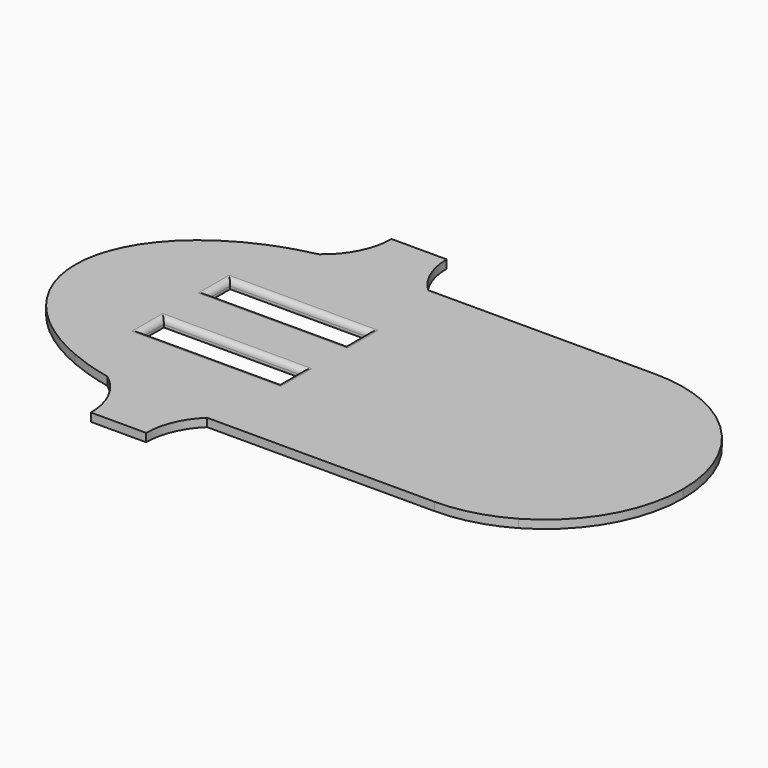
from build123d import *

# Parameters (mm, degrees)
F1_DEPTH = 3
F2_R     = 2
F3_DEPTH = 2


with BuildPart() as f1:
    # F0 (on Top) → F1 (new body)
    with BuildSketch(Plane.XY):
        with BuildLine():
            add(Edge.make_bspline(
                [(0, 0), (10.2976274735, 0), (20.158993222, 2.1182632902)],
                knots=[1.5707963268, 1.5707963268, 1.5707963268, 1.8629189995, 1.8629189995, 1.8629189995], degree=2, weights=[1, 0.9893519935, 1]))
            Line((0, 0), (17.6506484271, 0))
            ThreePointArc((17.6506484271, 0), (18.8700107709, 1.1003520247), (20.158993222, 2.1182632902))
        make_face()
        with BuildLine():
            add(Edge.make_bspline(
                [(-20.158993222, 2.1182632902), (-10.2976274735, 0), (0, 0)],
                knots=[1.2786736541, 1.2786736541, 1.2786736541, 1.5707963268, 1.5707963268, 1.5707963268], degree=2, weights=[1, 0.9893519935, 1]))
            Line((0, 0), (0, 30))
            Line((0, 30), (-10, 30))
            Line((-10, 30), (-30, 30))
            Line((-30, 30), (-30, 40))
            Line((-30, 40), (-10, 40))
            Line((-10, 40), (0, 40))
            Line((0, 40), (0, 50))
            Line((0, 50), (-70, 50))
            add(Edge.make_bspline(
                [(-70, 50), (-70, 21.516086051), (-35.6976035326, 6.9902650909)],
                knots=[0, 0, 0, 1.0356513364, 1.0356513364, 1.0356513364], degree=2, weights=[1, 0.8688975097, 1]))
            ThreePointArc((-35.6976035326, 6.9902650909), (-27.5204903752, 5.8549142898), (-20.158993222, 2.1182632902))
        make_face()
        with BuildLine():
            Line((0, -18), (0, 0))
            add(Edge.make_bspline(
                [(-20.158993222, 2.1182632902), (-10.2976274735, 0), (0, 0)],
                knots=[1.2786736541, 1.2786736541, 1.2786736541, 1.5707963268, 1.5707963268, 1.5707963268], degree=2, weights=[1, 0.9893519935, 1]))
            ThreePointArc((-20.158993222, 2.1182632902), (-12.6838044298, -6.7311307011), (-10, -18))
            Line((-10, -18), (0, -18))
        make_face()
        with BuildLine():
            Line((0, 30), (0, 0))
            add(Edge.make_bspline(
                [(0, 0), (10.2976274735, 0), (20.158993222, 2.1182632902)],
                knots=[1.5707963268, 1.5707963268, 1.5707963268, 1.8629189995, 1.8629189995, 1.8629189995], degree=2, weights=[1, 0.9893519935, 1]))
            ThreePointArc((20.158993222, 2.1182632902), (27.5204903752, 5.8549142898), (35.6976035326, 6.9902650909))
            add(Edge.make_bspline(
                [(35.6976035326, 6.9902650909), (49.4779363229, 12.8257362969), (58.3333333333, 22.3614600804)],
                knots=[2.1059413172, 2.1059413172, 2.1059413172, 2.5559071101, 2.5559071101, 2.5559071101], degree=2, weights=[1, 0.9747979228, 1]))
            ThreePointArc((58.3333333333, 22.3614600804), (52.1286446122, 35.5662432703), (50, 50))
            Line((50, 50), (0, 50))
            Line((0, 50), (0, 40))
            Line((0, 40), (20, 40))
            Line((20, 40), (20, 30))
            Line((20, 30), (0, 30))
        make_face()
        with BuildLine():
            Line((17.6506484271, 0), (0, 0))
            Line((0, 0), (0, -18))
            Line((0, -18), (10, -18))
            ThreePointArc((10, -18), (11.9920254116, -8.2207819669), (17.6506484271, 0))
        make_face()
        with BuildLine():
            ThreePointArc((20.158993222, 2.1182632902), (18.8700107709, 1.1003520247), (17.6506484271, 0))
            Line((17.6506484271, 0), (52.3493515729, 0))
            ThreePointArc((52.3493515729, 0), (44.67672975, 5.0512668056), (35.6976035326, 6.9902650909))
            add(Edge.make_bspline(
                [(20.158993222, 2.1182632902), (28.3447518468, 3.8765990461), (35.6976035326, 6.9902650909)],
                knots=[1.8629189995, 1.8629189995, 1.8629189995, 2.1059413172, 2.1059413172, 2.1059413172], degree=2, weights=[1, 0.9926265982, 1]))
        make_face()
        with BuildLine():
            add(Edge.make_bspline(
                [(-35.6976035326, 6.9902650909), (-28.3447518468, 3.8765990461), (-20.158993222, 2.1182632902)],
                knots=[1.0356513364, 1.0356513364, 1.0356513364, 1.2786736541, 1.2786736541, 1.2786736541], degree=2, weights=[1, 0.9926265982, 1]))
            ThreePointArc((-20.158993222, 2.1182632902), (-27.5204903752, 5.8549142898), (-35.6976035326, 6.9902650909))
        make_face()
        with BuildLine():
            ThreePointArc((35.6976035326, 6.9902650909), (27.5204903752, 5.8549142898), (20.158993222, 2.1182632902))
            add(Edge.make_bspline(
                [(20.158993222, 2.1182632902), (28.3447518468, 3.8765990461), (35.6976035326, 6.9902650909)],
                knots=[1.8629189995, 1.8629189995, 1.8629189995, 2.1059413172, 2.1059413172, 2.1059413172], degree=2, weights=[1, 0.9926265982, 1]))
        make_face()
        with BuildLine():
            ThreePointArc((35.6976035326, 6.9902650909), (44.67672975, 5.0512668056), (52.3493515729, 0))
            Line((52.3493515729, 0), (100, 0))
            ThreePointArc((100, 0), (76.3560472423, 5.9436327191), (58.3333333333, 22.3614600804))
            add(Edge.make_bspline(
                [(35.6976035326, 6.9902650909), (49.4779363229, 12.8257362969), (58.3333333333, 22.3614600804)],
                knots=[2.1059413172, 2.1059413172, 2.1059413172, 2.5559071101, 2.5559071101, 2.5559071101], degree=2, weights=[1, 0.9747979228, 1]))
        make_face()
        with BuildLine():
            ThreePointArc((58.3333333333, 22.3614600804), (76.3560472423, 5.9436327191), (100, 0))
            ThreePointArc((100, 0), (112.9409522551, 1.7037086855), (125, 6.6987298108))
            ThreePointArc((125, 6.6987298108), (110.8310397827, 18.9227968521), (102.1486677301, 35.5))
            Line((102.1486677301, 35.5), (85.5, 35.5))
            Line((85.5, 35.5), (85.5, 50))
            Line((85.5, 50), (70, 50))
            add(Edge.make_bspline(
                [(58.3333333333, 22.3614600804), (70, 34.9244327711), (70, 50)],
                knots=[2.5559071101, 2.5559071101, 2.5559071101, 3.1415926536, 3.1415926536, 3.1415926536], degree=2, weights=[1, 0.9574271078, 1]))
        make_face()
        with BuildLine():
            add(Edge.make_bspline(
                [(-35.6976035326, 93.0097349091), (-70, 78.483913949), (-70, 50)],
                knots=[5.2475339708, 5.2475339708, 5.2475339708, 6.2831853072, 6.2831853072, 6.2831853072], degree=2, weights=[1, 0.8688975097, 1]))
            Line((-70, 50), (0, 50))
            Line((0, 50), (0, 60))
            Line((0, 60), (-10, 60))
            Line((-10, 60), (-30, 60))
            Line((-30, 60), (-30, 70))
            Line((-30, 70), (-10, 70))
            Line((-10, 70), (0, 70))
            Line((0, 70), (0, 100))
            add(Edge.make_bspline(
                [(0, 100), (-10.2976274735, 100), (-20.158993222, 97.8817367098)],
                knots=[4.7123889804, 4.7123889804, 4.7123889804, 5.0045116531, 5.0045116531, 5.0045116531], degree=2, weights=[1, 0.9893519935, 1]))
            add(Edge.make_bspline(
                [(-20.158993222, 97.8817367098), (-28.3447518468, 96.1234009539), (-35.6976035326, 93.0097349091)],
                knots=[5.0045116531, 5.0045116531, 5.0045116531, 5.2475339708, 5.2475339708, 5.2475339708], degree=2, weights=[1, 0.9926265982, 1]))
        make_face()
        with BuildLine():
            ThreePointArc((50, 50), (52.1286446122, 35.5662432703), (58.3333333333, 22.3614600804))
            add(Edge.make_bspline(
                [(58.3333333333, 22.3614600804), (70, 34.9244327711), (70, 50)],
                knots=[2.5559071101, 2.5559071101, 2.5559071101, 3.1415926536, 3.1415926536, 3.1415926536], degree=2, weights=[1, 0.9574271078, 1]))
            Line((70, 50), (50, 50))
        make_face()
        with BuildLine():
            ThreePointArc((102.1486677301, 35.5), (110.8310397827, 18.9227968521), (125, 6.6987298108))
            ThreePointArc((125, 6.6987298108), (143.3012701892, 25), (150, 50))
            Line((150, 50), (114.5, 50))
            Line((114.5, 50), (114.5, 35.5))
            Line((114.5, 35.5), (102.1486677301, 35.5))
        make_face()
        with BuildLine():
            Line((0, 60), (0, 50))
            Line((0, 50), (50, 50))
            ThreePointArc((50, 50), (52.1286446122, 64.4337567297), (58.3333333333, 77.6385399196))
            add(Edge.make_bspline(
                [(58.3333333333, 77.6385399196), (49.4779363229, 87.1742637031), (35.6976035326, 93.0097349091)],
                knots=[3.727278197, 3.727278197, 3.727278197, 4.17724399, 4.17724399, 4.17724399], degree=2, weights=[1, 0.9747979228, 1]))
            ThreePointArc((35.6976035326, 93.0097349091), (27.5204903752, 94.1450857102), (20.158993222, 97.8817367098))
            add(Edge.make_bspline(
                [(20.158993222, 97.8817367098), (10.2976274735, 100), (0, 100)],
                knots=[4.4202663077, 4.4202663077, 4.4202663077, 4.7123889804, 4.7123889804, 4.7123889804], degree=2, weights=[1, 0.9893519935, 1]))
            Line((0, 100), (0, 70))
            Line((0, 70), (20, 70))
            Line((20, 70), (20, 60))
            Line((20, 60), (0, 60))
        make_face()
        with BuildLine():
            Line((50, 50), (70, 50))
            add(Edge.make_bspline(
                [(70, 50), (70, 65.0755672289), (58.3333333333, 77.6385399196)],
                knots=[3.1415926536, 3.1415926536, 3.1415926536, 3.727278197, 3.727278197, 3.727278197], degree=2, weights=[1, 0.9574271078, 1]))
            ThreePointArc((58.3333333333, 77.6385399196), (52.1286446122, 64.4337567297), (50, 50))
        make_face()
        with BuildLine():
            add(Edge.make_bspline(
                [(70, 50), (70, 65.0755672289), (58.3333333333, 77.6385399196)],
                knots=[3.1415926536, 3.1415926536, 3.1415926536, 3.727278197, 3.727278197, 3.727278197], degree=2, weights=[1, 0.9574271078, 1]))
            Line((70, 50), (85.5, 50))
            Line((85.5, 50), (85.5, 64.5))
            Line((85.5, 64.5), (102.1486677301, 64.5))
            ThreePointArc((102.1486677301, 64.5), (110.8310397827, 81.0772031479), (125, 93.3012701892))
            ThreePointArc((125, 93.3012701892), (112.9409522551, 98.2962913145), (100, 100))
            ThreePointArc((100, 100), (76.3560472423, 94.0563672809), (58.3333333333, 77.6385399196))
        make_face()
        with BuildLine():
            Line((85.5, 35.5), (102.1486677301, 35.5))
            ThreePointArc((102.1486677301, 35.5), (101.8578009321, 36.4970866512), (101.5877081724, 37.5))
            Line((101.5877081724, 37.5), (87.5, 37.5))
            Line((87.5, 37.5), (87.5, 50))
            Line((87.5, 50), (85.5, 50))
            Line((85.5, 50), (85.5, 35.5))
        make_face()
        with BuildLine():
            ThreePointArc((101.5877081724, 37.5), (101.8578009321, 36.4970866512), (102.1486677301, 35.5))
            Line((102.1486677301, 35.5), (114.5, 35.5))
            Line((114.5, 35.5), (114.5, 50))
            Line((114.5, 50), (112.5, 50))
            Line((112.5, 50), (112.5, 37.5))
            Line((112.5, 37.5), (101.5877081724, 37.5))
        make_face()
        with BuildLine():
            Line((114.5, 50), (150, 50))
            ThreePointArc((150, 50), (143.3012701892, 75), (125, 93.3012701892))
            ThreePointArc((125, 93.3012701892), (110.8310397827, 81.0772031479), (102.1486677301, 64.5))
            Line((102.1486677301, 64.5), (114.5, 64.5))
            Line((114.5, 64.5), (114.5, 50))
        make_face()
        with BuildLine():
            ThreePointArc((-10, 118), (-12.6838044298, 106.7311307011), (-20.158993222, 97.8817367098))
            add(Edge.make_bspline(
                [(0, 100), (-10.2976274735, 100), (-20.158993222, 97.8817367098)],
                knots=[4.7123889804, 4.7123889804, 4.7123889804, 5.0045116531, 5.0045116531, 5.0045116531], degree=2, weights=[1, 0.9893519935, 1]))
            Line((0, 100), (0, 118))
            Line((0, 118), (-10, 118))
        make_face()
        with BuildLine():
            add(Edge.make_bspline(
                [(58.3333333333, 77.6385399196), (49.4779363229, 87.1742637031), (35.6976035326, 93.0097349091)],
                knots=[3.727278197, 3.727278197, 3.727278197, 4.17724399, 4.17724399, 4.17724399], degree=2, weights=[1, 0.9747979228, 1]))
            ThreePointArc((58.3333333333, 77.6385399196), (76.3560472423, 94.0563672809), (100, 100))
            Line((100, 100), (52.3493515729, 100))
            ThreePointArc((52.3493515729, 100), (44.67672975, 94.9487331944), (35.6976035326, 93.0097349091))
        make_face()
        with BuildLine():
            Line((85.5, 64.5), (85.5, 50))
            Line((85.5, 50), (87.5, 50))
            Line((87.5, 50), (87.5, 62.5))
            Line((87.5, 62.5), (101.5877081724, 62.5))
            ThreePointArc((101.5877081724, 62.5), (101.8578009321, 63.5029133488), (102.1486677301, 64.5))
            Line((102.1486677301, 64.5), (85.5, 64.5))
        make_face()
        with BuildLine():
            Line((87.5, 37.5), (101.5877081724, 37.5))
            ThreePointArc((101.5877081724, 37.5), (100.3985151866, 43.6997853759), (100, 50))
            Line((100, 50), (87.5, 50))
            Line((87.5, 50), (87.5, 37.5))
        make_face()
        with BuildLine():
            ThreePointArc((100, 50), (100.3985151866, 43.6997853759), (101.5877081724, 37.5))
            Line((101.5877081724, 37.5), (112.5, 37.5))
            Line((112.5, 37.5), (112.5, 50))
            Line((112.5, 50), (100, 50))
        make_face()
        with BuildLine():
            Line((112.5, 50), (114.5, 50))
            Line((114.5, 50), (114.5, 64.5))
            Line((114.5, 64.5), (102.1486677301, 64.5))
            ThreePointArc((102.1486677301, 64.5), (101.8578009321, 63.5029133488), (101.5877081724, 62.5))
            Line((101.5877081724, 62.5), (112.5, 62.5))
            Line((112.5, 62.5), (112.5, 50))
        make_face()
        with BuildLine():
            Line((0, 118), (0, 100))
            Line((0, 100), (17.6506484271, 100))
            ThreePointArc((17.6506484271, 100), (11.9920254116, 108.2207819669), (10, 118))
            Line((10, 118), (0, 118))
        make_face()
        with BuildLine():
            Line((17.6506484271, 100), (0, 100))
            add(Edge.make_bspline(
                [(20.158993222, 97.8817367098), (10.2976274735, 100), (0, 100)],
                knots=[4.4202663077, 4.4202663077, 4.4202663077, 4.7123889804, 4.7123889804, 4.7123889804], degree=2, weights=[1, 0.9893519935, 1]))
            ThreePointArc((20.158993222, 97.8817367098), (18.8700107709, 98.8996479753), (17.6506484271, 100))
        make_face()
        with BuildLine():
            ThreePointArc((20.158993222, 97.8817367098), (27.5204903752, 94.1450857102), (35.6976035326, 93.0097349091))
            add(Edge.make_bspline(
                [(35.6976035326, 93.0097349091), (28.3447518468, 96.1234009539), (20.158993222, 97.8817367098)],
                knots=[4.17724399, 4.17724399, 4.17724399, 4.4202663077, 4.4202663077, 4.4202663077], degree=2, weights=[1, 0.9926265982, 1]))
        make_face()
        with BuildLine():
            add(Edge.make_bspline(
                [(35.6976035326, 93.0097349091), (28.3447518468, 96.1234009539), (20.158993222, 97.8817367098)],
                knots=[4.17724399, 4.17724399, 4.17724399, 4.4202663077, 4.4202663077, 4.4202663077], degree=2, weights=[1, 0.9926265982, 1]))
            ThreePointArc((35.6976035326, 93.0097349091), (44.67672975, 94.9487331944), (52.3493515729, 100))
            Line((52.3493515729, 100), (17.6506484271, 100))
            ThreePointArc((17.6506484271, 100), (18.8700107709, 98.8996479753), (20.158993222, 97.8817367098))
        make_face()
        with BuildLine():
            Line((87.5, 62.5), (87.5, 50))
            Line((87.5, 50), (100, 50))
            ThreePointArc((100, 50), (100.3985151866, 56.3002146241), (101.5877081724, 62.5))
            Line((101.5877081724, 62.5), (87.5, 62.5))
        make_face()
        with BuildLine():
            ThreePointArc((101.5877081724, 62.5), (100.3985151866, 56.3002146241), (100, 50))
            Line((100, 50), (112.5, 50))
            Line((112.5, 50), (112.5, 62.5))
            Line((112.5, 62.5), (101.5877081724, 62.5))
        make_face()
    extrude(amount=F1_DEPTH)

    # F2
    f2_edges = [f1.edges().sort_by_distance(p)[0] for p in [
        (20, 65, 3),
        (20, 35, 3),
        (-5, 40, 3),
        (-5, 60, 3),
        (-5, 30, 3),
        (-30, 35, 3),
        (-30, 65, 3),
        (-5, 70, 3),
    ]]
    fillet(f2_edges, radius=F2_R)

    # F0 (on Top) → F3 (join)
    with BuildSketch(Plane.XY):
        with BuildLine():
            Line((85.5, 35.5), (102.1486677301, 35.5))
            ThreePointArc((102.1486677301, 35.5), (101.8578009321, 36.4970866512), (101.5877081724, 37.5))
            Line((101.5877081724, 37.5), (87.5, 37.5))
            Line((87.5, 37.5), (87.5, 50))
            Line((87.5, 50), (85.5, 50))
            Line((85.5, 50), (85.5, 35.5))
        make_face()
        with BuildLine():
            ThreePointArc((101.5877081724, 37.5), (101.8578009321, 36.4970866512), (102.1486677301, 35.5))
            Line((102.1486677301, 35.5), (114.5, 35.5))
            Line((114.5, 35.5), (114.5, 50))
            Line((114.5, 50), (112.5, 50))
            Line((112.5, 50), (112.5, 37.5))
            Line((112.5, 37.5), (101.5877081724, 37.5))
        make_face()
        with BuildLine():
            Line((112.5, 50), (114.5, 50))
            Line((114.5, 50), (114.5, 64.5))
            Line((114.5, 64.5), (102.1486677301, 64.5))
            ThreePointArc((102.1486677301, 64.5), (101.8578009321, 63.5029133488), (101.5877081724, 62.5))
            Line((101.5877081724, 62.5), (112.5, 62.5))
            Line((112.5, 62.5), (112.5, 50))
        make_face()
        with BuildLine():
            Line((85.5, 64.5), (85.5, 50))
            Line((85.5, 50), (87.5, 50))
            Line((87.5, 50), (87.5, 62.5))
            Line((87.5, 62.5), (101.5877081724, 62.5))
            ThreePointArc((101.5877081724, 62.5), (101.8578009321, 63.5029133488), (102.1486677301, 64.5))
            Line((102.1486677301, 64.5), (85.5, 64.5))
        make_face()
    extrude(amount=-F3_DEPTH)


solid = f1.part
